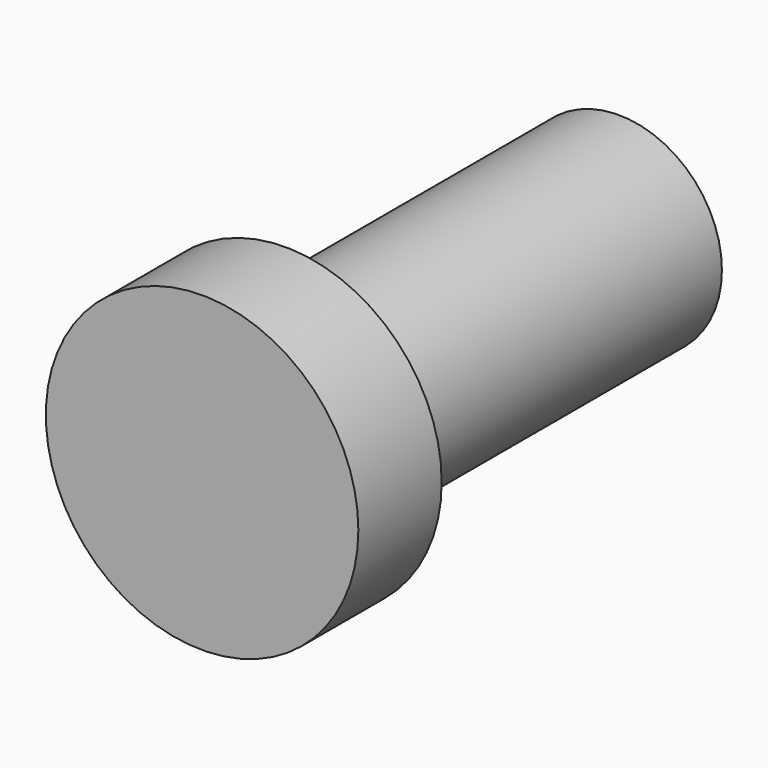
from build123d import *
from build123d import SkipClean  # not in build123d's __all__

# Parameters (mm, degrees)
F0_R     = 0.495
F1_DEPTH = 2
F2_R     = 0.75
F2_R_2   = 0.495
F3_DEPTH = 0.5


with BuildPart() as f1:
    # F0 (on Front) → F1 (new body)
    with BuildSketch(Plane.XZ):
        Circle(F0_R)
    extrude(amount=F1_DEPTH)

    # F2 (on face) → F3 (join)
    with BuildSketch(Plane.XZ.offset(2)):
        Circle(F2_R)
        Circle(F2_R_2, mode=Mode.SUBTRACT)
        Circle(F2_R_2)
    extrude(amount=F3_DEPTH)

    # F4 (on Right) → F5 (revolve, cut)
    with BuildSketch(Plane.YZ):
        with BuildLine():
            Line((0.25, 0), (0.25, 0.5))
            ThreePointArc((0.25, 0.5), (-0.25, 0), (0.25, -0.5))
            Line((0.25, -0.5), (0.25, 0))
        make_face()
    with SkipClean():  # cleaning this boolean's faces spoils the solid; the shape is the same uncleaned
        revolve(axis=Axis((0, 0.25, 0.25), (0, 0, 1)), mode=Mode.SUBTRACT)


solid = f1.part
